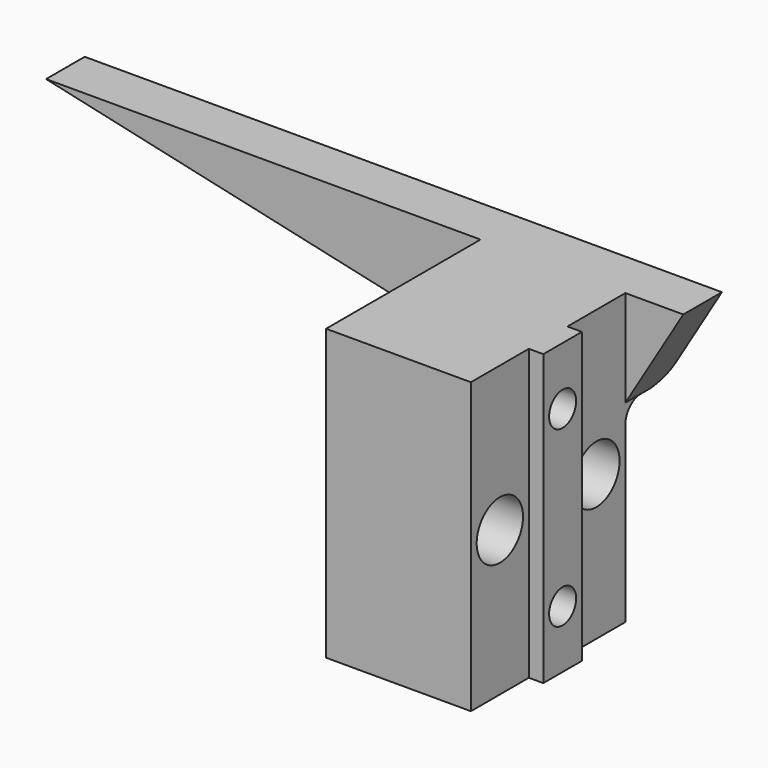
from build123d import *

# Parameters (mm, degrees)
F1_DEPTH     = 30
F2_R         = 1.75
F3_DEPTH     = 16.501
F4_R         = 3
F5_DEPTH     = 13
F6_R         = 3
F7_DEPTH     = 13
F9_DEPTH     = 5
F10_T1_DEPTH = 15
F10_T3_DEPTH = 35


# Not quite as in the source:
# - a fillet or chamfer that OpenCascade refuses, or shapes differently, is made with other operations: its cross-section is extruded or revolved along the edge and cut away or added


with BuildPart() as f1:
    # F0 (on Top) → F1 (new body)
    with BuildSketch(Plane.XY):
        Polygon((0, -7.5), (0, 0), (-15, 0), (-15, -20), (0, -20), (0, -12.5), (1.5, -12.5), (1.5, -7.5), align=None)
    extrude(amount=F1_DEPTH)

    # F2 (on face) → F3 (cut, through all)
    with BuildSketch(Plane(origin=(-15, 0, 0), x_dir=(0, -1, 0), z_dir=(-1, 0, 0))):
        with Locations((10, 24)):
            Circle(F2_R)
        with Locations((10, 6)):
            Circle(F2_R)
    extrude(amount=-F3_DEPTH, mode=Mode.SUBTRACT)

    # F4 (on face) → F5 (cut)
    with BuildSketch(Plane.YZ):
        with Locations((-16.25, 15)):
            Circle(F4_R)
    extrude(amount=-F5_DEPTH, mode=Mode.SUBTRACT)

    # F6 (on face) → F7 (cut)
    with BuildSketch(Plane.YZ):
        with Locations((-3.75, 15)):
            Circle(F6_R)
    extrude(amount=-F7_DEPTH, mode=Mode.SUBTRACT)

    # F8 (on face) → F9 (join)
    with BuildSketch(Plane(origin=(0, 0, 0), x_dir=(-1, 0, 0), z_dir=(0, 1, 0))):
        Polygon((60, 30), (15, 30), (-6, 30), (0, 20), (15, 20), align=None)
    extrude(amount=F9_DEPTH)

    # F10: fillet of radius 2 on 2 edges, made by hand

    # F10_s2 → F10_t1 (join)
    with BuildSketch(Plane.YZ.offset(-15)):
        with BuildLine():
            ThreePointArc((0, 18), (0.5857864376, 19.4142135624), (2, 20))
            Line((2, 20), (0, 20))
            Line((0, 20), (0, 18))
        make_face()
    extrude(amount=F10_T1_DEPTH)

    # F10_s4 → F10_t3 (cut)
    with BuildSketch(Plane.YZ.offset(-30)):
        with BuildLine():
            ThreePointArc((5, 22), (4.4142135624, 20.5857864376), (3, 20))
            Line((3, 20), (5, 20))
            Line((5, 20), (5, 22))
        make_face()
    extrude(amount=F10_T3_DEPTH, mode=Mode.SUBTRACT)


solid = f1.part
